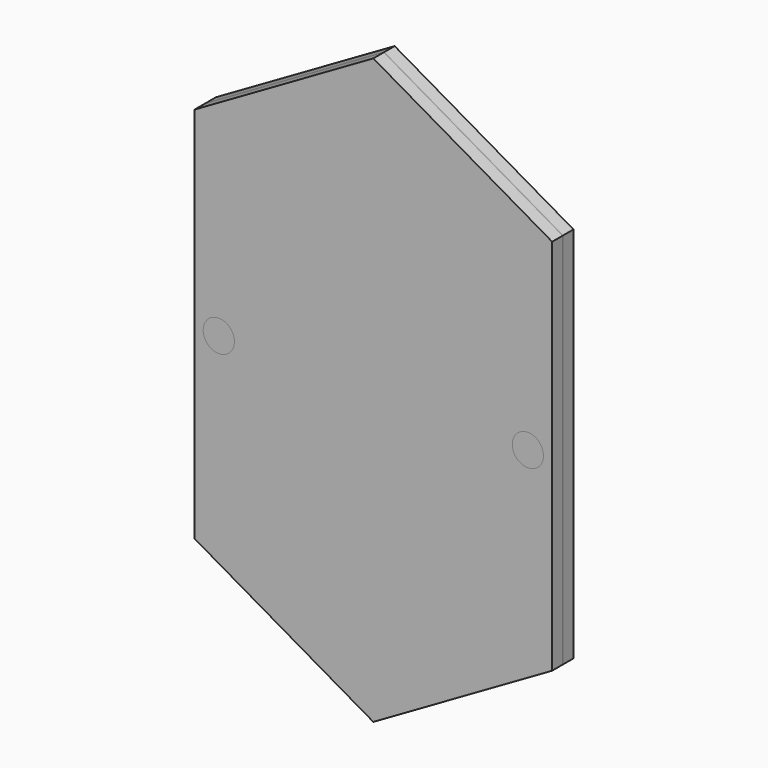
from build123d import *

# Parameters (mm, degrees)
F1_DEPTH = 0.1
F3_DEPTH = 4
F4_R     = 4.8
F5_DEPTH = 1.6
F7_R     = 4.8
F8_DEPTH = 1.6


# Not quite as in the source:
# - a feature names something its author has since deleted; it is built from what else it names


with BuildPart() as f1:
    # F0 (on Front) → F1 (new body, symmetric)
    with BuildSketch(Plane.XZ):
        Polygon((-55, 31.7542648054), (0, 0), (55, 31.7542648054), (55, 147.9135872183), (0, 179.6678520237), (-55, 147.9135872183), align=None)
    extrude(amount=F1_DEPTH, both=True)

    # F4 (on face) → F5 (cut)
    with BuildSketch(Plane.XZ.offset(4.1)):
        with Locations((62, 89.8339260119)):
            Circle(F4_R)
        with Locations((-62, 89.8339260119)):
            Circle(F4_R)
    extrude(amount=-F5_DEPTH, mode=Mode.SUBTRACT)


with BuildPart() as f3:
    # F2 (on face) → F3 (new body)
    with BuildSketch(Plane.XZ.offset(0.1)):
        Polygon((0, 179.6678520237), (-55, 147.9135872183), (-55, 31.7542648054), (0, 0), (55, 31.7542648054), (55, 147.9135872183), align=None)
    extrude(amount=F3_DEPTH)


with BuildPart() as f6_1:
    # F6: instance of F3
    add(f3.part.mirror(Plane.XZ))


with BuildPart() as f8:
    # F7 (on face) → F8 (new body)
    with BuildSketch(Plane.XZ.offset(4.1)):
        with Locations((-47.5324755942, 89.0702977777)):
            Circle(F7_R)
    extrude(amount=-F8_DEPTH)


with BuildPart() as f8b:
    # F7 (on face) → F8, piece 2 (new body)
    with BuildSketch(Plane.XZ.offset(4.1)):
        with Locations((47.5324755942, 89.0702977777)):
            Circle(F7_R)
    extrude(amount=-F8_DEPTH)


solid = Compound([f1.part, f3.part, f6_1.part, f8.part, f8b.part])
